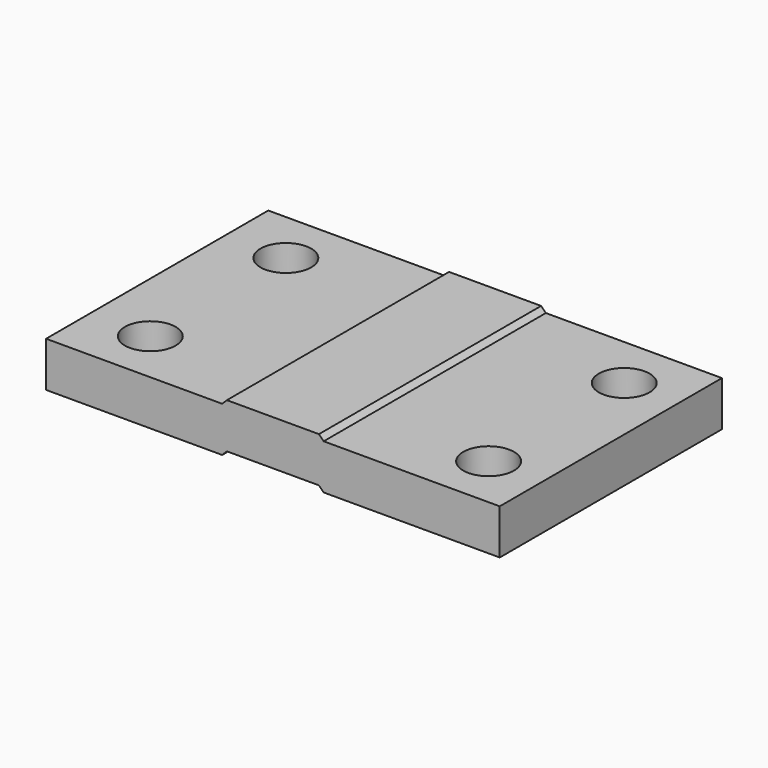
from build123d import *

# Parameters (mm, degrees)
F1_DEPTH = 13.32
F4_DEPTH = 82.081
F7_DEPTH = 82.08
F9_D     = 15


with BuildPart() as f1:
    # F0 (on Top) → F1 (new body)
    with BuildSketch(Plane.XY):
        Polygon((-67.04, 0), (0, 0), (67.04, 0), (67.04, 82.08), (-67.04, 82.08), align=None)
    extrude(amount=F1_DEPTH)

    # F3 (on offset) → F4 (cut, through all)
    with BuildSketch(Plane.XZ):
        Polygon((-15, 0), (0, 0), (15, 0), (13.6, 1.4), (-13.6, 1.4), align=None)
    extrude(amount=-F4_DEPTH, mode=Mode.SUBTRACT)

    # F6 (on offset) → F7 (join)
    with BuildSketch(Plane.XZ):
        Polygon((-15, 13.32), (0, 13.32), (15, 13.32), (13.6, 14.72), (-13.6, 14.72), align=None)
    extrude(amount=-F7_DEPTH)

    # F9 (through all)
    with Locations(Plane(origin=(0, 0, 0), x_dir=(1, 0, 0), z_dir=(0, 0, -1))):
        with Locations((-49.04, -66.08), (-49.04, -16), (50.96, -16), (50.96, -66.08)):
            Hole(F9_D / 2)


solid = f1.part
